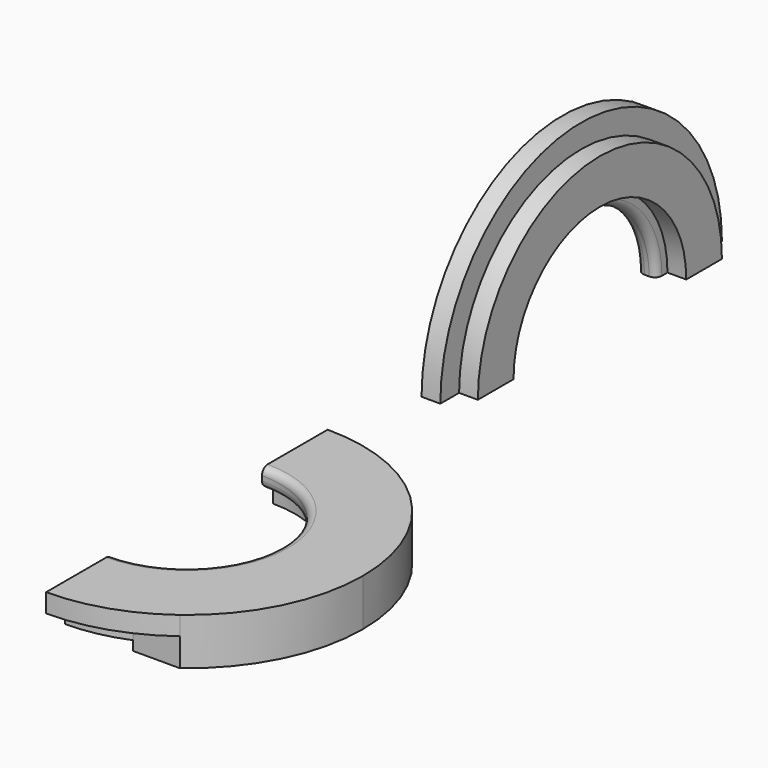
from build123d import *

# Parameters (mm, degrees)
F1_DEPTH  = 2
F2_DEPTH  = 3
F3_DEPTH  = 2
F5_DEPTH  = 4
F6_DEPTH  = 2
F8_DEPTH  = 2
F9_R      = 0.75
F11_DEPTH = 2
F12_R     = 0.75


with BuildPart() as f1:
    # F0 (on Top) → F1 (new body)
    with BuildSketch(Plane.XY):
        with BuildLine():
            ThreePointArc((0, 16.25), (3.186887196, 15.93443598), (6.25, 15))
            Line((6.25, 15), (11.25, 15))
            ThreePointArc((11.25, 15), (5.9292706128, 17.7878118384), (0, 18.75))
            Line((0, 18.75), (0, 16.25))
        make_face()
        with BuildLine():
            ThreePointArc((6.25, 15), (13.520817283, 9.0138781887), (16.25, 0))
            ThreePointArc((16.25, 0), (13.520817283, -9.0138781887), (6.25, -15))
            Line((6.25, -15), (11.25, -15))
            ThreePointArc((11.25, -15), (16.7705098312, -8.3852549156), (18.75, 0))
            ThreePointArc((18.75, 0), (16.7705098312, 8.3852549156), (11.25, 15))
            Line((11.25, 15), (6.25, 15))
        make_face()
        with BuildLine():
            Line((11.25, -15), (6.25, -15))
            ThreePointArc((6.25, -15), (3.186887196, -15.93443598), (0, -16.25))
            Line((0, -16.25), (0, -18.75))
            ThreePointArc((0, -18.75), (5.9292706128, -17.7878118384), (11.25, -15))
        make_face()
        with BuildLine():
            ThreePointArc((6.25, -15), (13.520817283, -9.0138781887), (16.25, 0))
            ThreePointArc((16.25, 0), (13.520817283, 9.0138781887), (6.25, 15))
            ThreePointArc((6.25, 15), (3.186887196, 15.93443598), (0, 16.25))
            Line((0, 16.25), (0, 10))
            ThreePointArc((0, 10), (7.0710678119, 7.0710678119), (10, 0))
            ThreePointArc((10, 0), (7.0710678119, -7.0710678119), (0, -10))
            Line((0, -10), (0, -16.25))
            ThreePointArc((0, -16.25), (3.186887196, -15.93443598), (6.25, -15))
        make_face()
    extrude(amount=F1_DEPTH)

    # F0 (on Top) → F2 (join)
    with BuildSketch(Plane.XY):
        with BuildLine():
            ThreePointArc((6.25, 15), (13.520817283, 9.0138781887), (16.25, 0))
            ThreePointArc((16.25, 0), (13.520817283, -9.0138781887), (6.25, -15))
            Line((6.25, -15), (11.25, -15))
            ThreePointArc((11.25, -15), (16.7705098312, -8.3852549156), (18.75, 0))
            ThreePointArc((18.75, 0), (16.7705098312, 8.3852549156), (11.25, 15))
            Line((11.25, 15), (6.25, 15))
        make_face()
    extrude(amount=-F2_DEPTH)

    # F0 (on Top) → F3 (join)
    with BuildSketch(Plane.XY):
        with BuildLine():
            ThreePointArc((6.25, -15), (13.520817283, -9.0138781887), (16.25, 0))
            ThreePointArc((16.25, 0), (13.520817283, 9.0138781887), (6.25, 15))
            ThreePointArc((6.25, 15), (3.186887196, 15.93443598), (0, 16.25))
            Line((0, 16.25), (0, 10))
            ThreePointArc((0, 10), (7.0710678119, 7.0710678119), (10, 0))
            ThreePointArc((10, 0), (7.0710678119, -7.0710678119), (0, -10))
            Line((0, -10), (0, -16.25))
            ThreePointArc((0, -16.25), (3.186887196, -15.93443598), (6.25, -15))
        make_face()
    extrude(amount=-F3_DEPTH)

    # F10 (on face) → F11 (cut)
    with BuildSketch(Plane(origin=(0, 0, -2), x_dir=(1, 0, 0), z_dir=(0, 0, -1))):
        with BuildLine():
            Line((0, -10), (0, -11.5))
            ThreePointArc((0, -11.5), (11.5, 0), (0, 11.5))
            Line((0, 11.5), (0, 10))
            ThreePointArc((0, 10), (10, 0), (0, -10))
        make_face()
    extrude(amount=-F11_DEPTH, mode=Mode.SUBTRACT)

    # F12
    f12_edges = [f1.edges().sort_by_distance(p)[0] for p in [
        (10, 0, 0),
        (10, 0, 2),
    ]]
    fillet(f12_edges, radius=F12_R)


with BuildPart() as f5:
    # F4 (on Right) → F5 (new body)
    with BuildSketch(Plane.YZ):
        with BuildLine():
            Line((60, 0), (66.25, 0))
            ThreePointArc((66.25, 0), (50, 16.25), (33.75, 0))
            Line((33.75, 0), (40, 0))
            ThreePointArc((40, 0), (50, 10), (60, 0))
        make_face()
    extrude(amount=F5_DEPTH)

    # F4 (on Right) → F6 (join)
    with BuildSketch(Plane.YZ):
        with BuildLine():
            Line((66.25, 0), (68.75, 0))
            ThreePointArc((68.75, 0), (50, 18.75), (31.25, 0))
            Line((31.25, 0), (33.75, 0))
            ThreePointArc((33.75, 0), (50, 16.25), (66.25, 0))
        make_face()
    extrude(amount=F6_DEPTH)

    # F7 (on face) → F8 (cut)
    with BuildSketch(Plane.YZ.offset(4)):
        with BuildLine():
            Line((60, 0), (61.5, 0))
            ThreePointArc((61.5, 0), (50, 11.5), (38.5, 0))
            Line((38.5, 0), (40, 0))
            ThreePointArc((40, 0), (50, 10), (60, 0))
        make_face()
    extrude(amount=-F8_DEPTH, mode=Mode.SUBTRACT)

    # F9
    f9_edges = [f5.edges().sort_by_distance(p)[0] for p in [
        (0, 50, 10),
        (2, 50, 10),
    ]]
    fillet(f9_edges, radius=F9_R)


solid = Compound([f1.part, f5.part])
